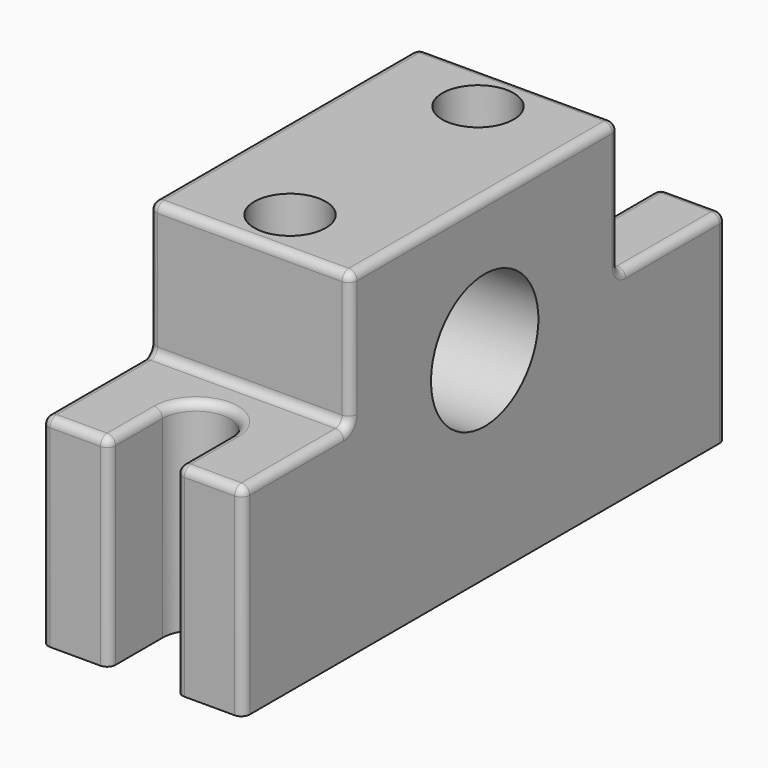
from build123d import *

# Parameters (mm, degrees)
F0_W     = 19.05
F0_H     = 6.35
F0_H_2   = 15.875
F0_R     = 3.571875
F0_H_3   = 9.525
F1_DEPTH = 19.05
F2_DEPTH = 31.75
F4_D     = 12.7
F6_D     = 6.7564
F6_DEPTH = 12.7
F6_TIP   = 2.0298273432
F7_R     = 0.79375


with BuildPart() as f1:
    # F0 (on Top) → F1 (new body)
    with BuildSketch(Plane.XY):
        with Locations((0, 3.175)):
            Rectangle(F0_W, F0_H)
        with BuildLine():
            Line((9.525, -28.575), (9.525, -15.875))
            Line((9.525, -15.875), (-9.525, -15.875))
            Line((-9.525, -15.875), (-9.525, -28.575))
            Line((-9.525, -28.575), (-3.175, -28.575))
            Line((-3.175, -28.575), (-3.175, -22.225))
            ThreePointArc((-3.175, -22.225), (0, -19.05), (3.175, -22.225))
            Line((3.175, -22.225), (3.175, -28.575))
            Line((3.175, -28.575), (9.525, -28.575))
        make_face()
        with Locations((0, -7.9375)):
            Rectangle(F0_W, F0_H_2)
        with Locations((0, -11.1125)):
            Circle(F0_R, mode=Mode.SUBTRACT)
        with Locations((0, 11.1125)):
            Rectangle(F0_W, F0_H_3)
        with Locations((0, 11.1125)):
            Circle(F0_R, mode=Mode.SUBTRACT)
        with BuildLine():
            Line((9.525, 15.875), (9.525, 28.575))
            Line((9.525, 28.575), (3.175, 28.575))
            Line((3.175, 28.575), (3.175, 22.225))
            ThreePointArc((3.175, 22.225), (0, 19.05), (-3.175, 22.225))
            Line((-3.175, 22.225), (-3.175, 28.575))
            Line((-3.175, 28.575), (-9.525, 28.575))
            Line((-9.525, 28.575), (-9.525, 15.875))
            Line((-9.525, 15.875), (9.525, 15.875))
        make_face()
        with Locations((0, 11.1125)):
            Circle(F0_R)
        with Locations((0, -11.1125)):
            Circle(F0_R)
    extrude(amount=F1_DEPTH)

    # F0 (on Top) → F2 (join)
    with BuildSketch(Plane.XY):
        with Locations((0, 3.175)):
            Rectangle(F0_W, F0_H)
        with Locations((0, -7.9375)):
            Rectangle(F0_W, F0_H_2)
        with Locations((0, -11.1125)):
            Circle(F0_R, mode=Mode.SUBTRACT)
        with Locations((0, 11.1125)):
            Rectangle(F0_W, F0_H_3)
        with Locations((0, 11.1125)):
            Circle(F0_R, mode=Mode.SUBTRACT)
        with Locations((0, -11.1125)):
            Circle(F0_R)
        with Locations((0, 11.1125)):
            Circle(F0_R)
    extrude(amount=F2_DEPTH)

    # F4 (through all)
    with Locations(Plane.YZ.offset(9.525)):
        with Locations((0, 19.05)):
            Hole(F4_D / 2)

    # F6
    with Locations(Plane.XY.offset(31.75)):
        with Locations((0, 11.1125), (0, -11.1125)):
            Hole(F6_D / 2, depth=F6_DEPTH)
            with Locations((0, 0, -(F6_DEPTH + F6_TIP / 2))):  # 118° drill point
                Cone(0, F6_D / 2, F6_TIP, mode=Mode.SUBTRACT)

    # F7
    f7_edges = [f1.edges().sort_by_distance(p)[0] for p in [
        (-9.525, 0, 31.75),
        (0, -15.875, 31.75),
        (9.525, 0, 31.75),
        (0, 15.875, 31.75),
        (9.525, 15.875, 25.4),
        (-9.525, 15.875, 25.4),
        (0, 15.875, 19.05),
        (9.525, 22.225, 19.05),
        (9.525, 28.575, 9.525),
        (-9.525, 28.575, 9.525),
        (6.35, 28.575, 19.05),
        (-6.35, 28.575, 19.05),
        (3.175, 28.575, 9.525),
        (-3.175, 28.575, 9.525),
        (3.175, 25.4, 19.05),
        (0, -15.875, 19.05),
        (9.525, -15.875, 25.4),
        (9.525, -22.225, 19.05),
        (-9.525, -22.225, 19.05),
        (-9.525, -15.875, 25.4),
        (-3.175, -25.4, 19.05),
        (6.35, -28.575, 19.05),
        (-6.35, -28.575, 19.05),
        (9.525, -28.575, 9.525),
        (-9.525, -28.575, 9.525),
        (3.175, -28.575, 9.525),
        (-3.175, -28.575, 9.525),
        (-9.525, 22.225, 19.05),
        (3.175, -25.4, 19.05),
        (0, -19.05, 19.05),
        (-3.175, 25.4, 19.05),
        (0, 19.05, 19.05),
    ]]
    fillet(f7_edges, radius=F7_R)


solid = f1.part
